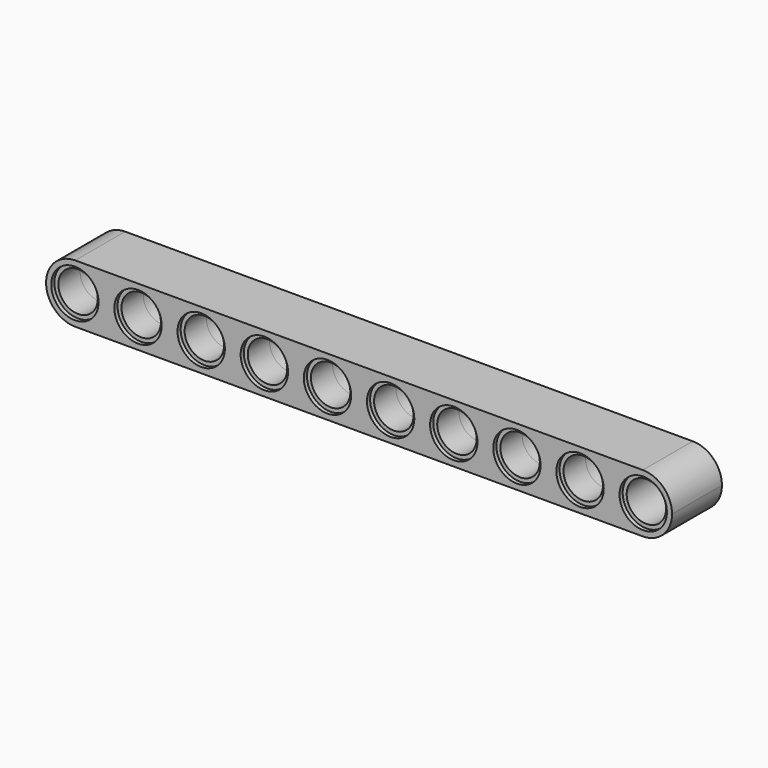
from build123d import *

# Parameters (mm, degrees)
F0_W     = 79.3
F0_H     = 7.4
F0_R     = 3
F1_DEPTH = 3.95
F0_R_2   = 2.499
F2_DEPTH = 3.45
F3_R     = 3.69999


# Not quite as in the source:
# - a fillet or chamfer is up to 0.001 mm smaller than in the source, because OpenCascade refuses the exact size


with BuildPart() as f1:
    # F0 (on Front) → F1 (new body, symmetric)
    with BuildSketch(Plane.XZ):
        with Locations((-4, 0)):
            Rectangle(F0_W, F0_H)
        with Locations((-40, 0)):
            Circle(F0_R, mode=Mode.SUBTRACT)
        with Locations((-32, 0)):
            Circle(F0_R, mode=Mode.SUBTRACT)
        with Locations((-24, 0)):
            Circle(F0_R, mode=Mode.SUBTRACT)
        with Locations((-16, 0)):
            Circle(F0_R, mode=Mode.SUBTRACT)
        with Locations((-8, 0)):
            Circle(F0_R, mode=Mode.SUBTRACT)
        Circle(F0_R, mode=Mode.SUBTRACT)
        with Locations((8, 0)):
            Circle(F0_R, mode=Mode.SUBTRACT)
        with Locations((16, 0)):
            Circle(F0_R, mode=Mode.SUBTRACT)
        with Locations((24, 0)):
            Circle(F0_R, mode=Mode.SUBTRACT)
        with Locations((32, 0)):
            Circle(F0_R, mode=Mode.SUBTRACT)
    extrude(amount=F1_DEPTH, both=True)

    # F0 (on Front) → F2 (join, symmetric)
    with BuildSketch(Plane.XZ):
        with Locations((-40, 0)):
            Circle(F0_R)
        with Locations((-40, 0)):
            Circle(F0_R_2, mode=Mode.SUBTRACT)
        with Locations((-32, 0)):
            Circle(F0_R)
        with Locations((-32, 0)):
            Circle(F0_R_2, mode=Mode.SUBTRACT)
        with Locations((-24, 0)):
            Circle(F0_R)
        with Locations((-24, 0)):
            Circle(F0_R_2, mode=Mode.SUBTRACT)
        with Locations((-16, 0)):
            Circle(F0_R)
        with Locations((-16, 0)):
            Circle(F0_R_2, mode=Mode.SUBTRACT)
        with Locations((-8, 0)):
            Circle(F0_R)
        with Locations((-8, 0)):
            Circle(F0_R_2, mode=Mode.SUBTRACT)
        Circle(F0_R)
        Circle(F0_R_2, mode=Mode.SUBTRACT)
        with Locations((8, 0)):
            Circle(F0_R)
        with Locations((8, 0)):
            Circle(F0_R_2, mode=Mode.SUBTRACT)
        with Locations((16, 0)):
            Circle(F0_R)
        with Locations((16, 0)):
            Circle(F0_R_2, mode=Mode.SUBTRACT)
        with Locations((24, 0)):
            Circle(F0_R)
        with Locations((24, 0)):
            Circle(F0_R_2, mode=Mode.SUBTRACT)
        with Locations((32, 0)):
            Circle(F0_R)
        with Locations((32, 0)):
            Circle(F0_R_2, mode=Mode.SUBTRACT)
    extrude(amount=F2_DEPTH, both=True)

    # F3 (radius 3.7 in the source; OpenCascade refuses exactly that, so slightly less here)
    f3_edges = [f1.edges().sort_by_distance(p)[0] for p in [
        (-43.65, 0, 3.7),
        (35.65, 0, 3.7),
        (35.65, 0, -3.7),
        (-43.65, 0, -3.7),
    ]]
    fillet(f3_edges, radius=F3_R)


solid = f1.part
